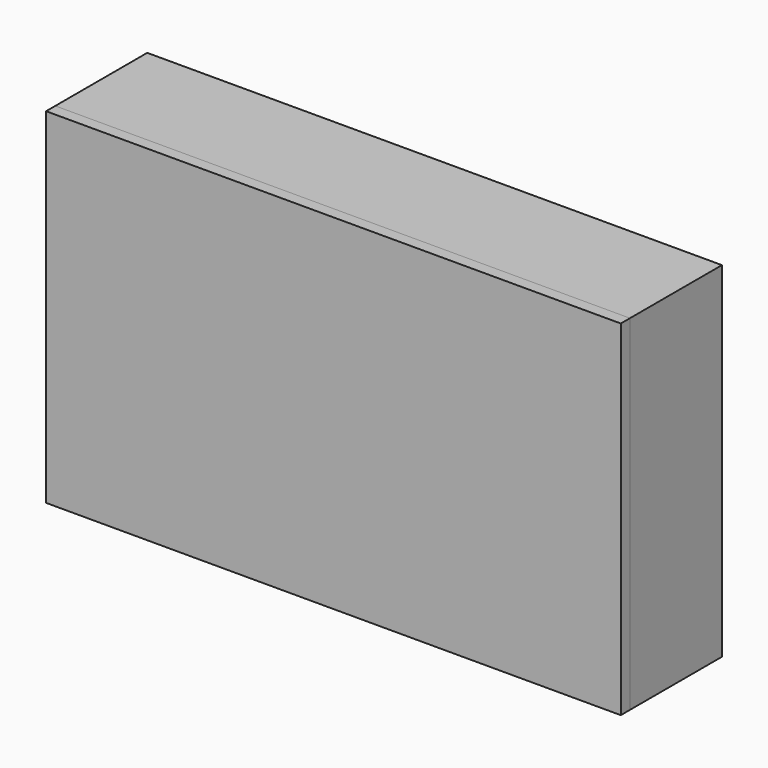
from build123d import *

# Parameters (mm, degrees)
F4_W     = 127
F4_H     = 76.2
F5_DEPTH = 25.4
F6_T     = -2.54
F0_W     = 121.92
F0_H     = 71.12
F0_W_2   = 116.84
F0_H_2   = 66.04
F1_DEPTH = 12.7
F2_DEPTH = 10.16
F3_W     = 127
F3_H     = 76.2
F7_DEPTH = 2.54


with BuildPart() as f5:
    # F4 (on Front) → F5 (new body)
    with BuildSketch(Plane.XZ):
        Rectangle(F4_W, F4_H)
    extrude(amount=F5_DEPTH)

    # F6
    f6_openings = [f5.faces().sort_by_distance(p)[0] for p in [
        (0, -25.4, 0),
    ]]
    offset(amount=F6_T, openings=f6_openings)

    # F0 (on face) → F1 (join)
    with BuildSketch(Plane.XZ.offset(2.54)):
        Rectangle(F0_W, F0_H)
        Rectangle(F0_W_2, F0_H_2, mode=Mode.SUBTRACT)
    extrude(amount=F1_DEPTH)


with BuildPart() as f2:
    # F2 (new): a face of the model
    f2_faces = [f5.part.faces().sort_by_distance(p)[0] for p in [
        (59.5485276907, -15.24, 0),
    ]]
    extrude(f2_faces, amount=F2_DEPTH)

    # F3 (on face) → F7 (join)
    with BuildSketch(Plane.XZ.offset(25.4)):
        Rectangle(F3_W, F3_H)
    extrude(amount=F7_DEPTH)


solid = Compound([f5.part, f2.part])
